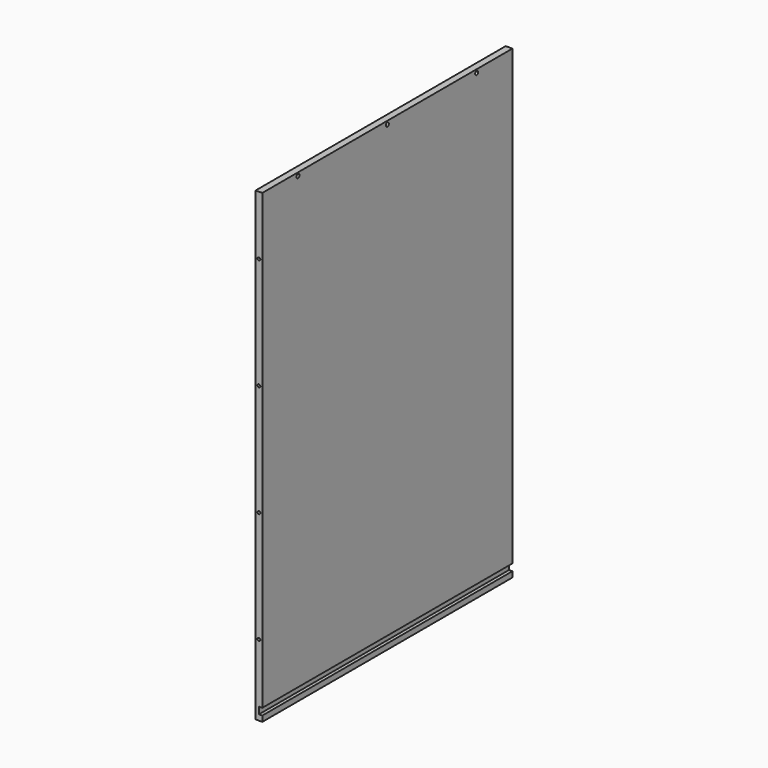
from build123d import *

# Parameters (mm, degrees)
F0_W     = 280
F0_H     = 417
F1_DEPTH = 6
F3_D     = 3.4
F4_W     = 280
F4_H     = 6.1
F5_DEPTH = 3
F8_D     = 2.5
F8_DEPTH = 16.5
F8_TIP   = 0.7510757738
F9_D     = 2.5
F9_DEPTH = 16.5
F9_TIP   = 0.7510757738


# Not quite as in the source:
# - a feature names something its author has since deleted; it is built from what else it names


with BuildPart() as f1:
    # F0 (on Right) → F1 (new body)
    with BuildSketch(Plane.YZ):
        Rectangle(F0_W, F0_H)
    extrude(amount=F1_DEPTH)

    # F3 (through all)
    with Locations(Plane.YZ.offset(6)):
        with Locations((100, 205.5), (0, 205.5), (-100, 205.5)):
            Hole(F3_D / 2)


with BuildPart() as f5:
    # F4 (on face) → F5 (new body)
    with BuildSketch(Plane.YZ.offset(6)):
        with Locations((0, -200.45)):
            Rectangle(F4_W, F4_H)
    extrude(amount=-F5_DEPTH)


with BuildPart() as f1_1:
    add(f1.part)

    # F6: cut F5
    add(f5.part, mode=Mode.SUBTRACT)

    # F8
    with Locations(Plane.XZ.offset(140)):
        with Locations((3, 155.5), (3, 55.5), (3, -44.5)):
            Hole(F8_D / 2, depth=F8_DEPTH)
            with Locations((0, 0, -(F8_DEPTH + F8_TIP / 2))):  # 118° drill point
                Cone(0, F8_D / 2, F8_TIP, mode=Mode.SUBTRACT)

    # F9
    with Locations(Plane.XZ.offset(140)):
        with Locations((3, -144.5)):
            Hole(F9_D / 2, depth=F9_DEPTH)
            with Locations((0, 0, -(F9_DEPTH + F9_TIP / 2))):  # 118° drill point
                Cone(0, F9_D / 2, F9_TIP, mode=Mode.SUBTRACT)


solid = f1_1.part
